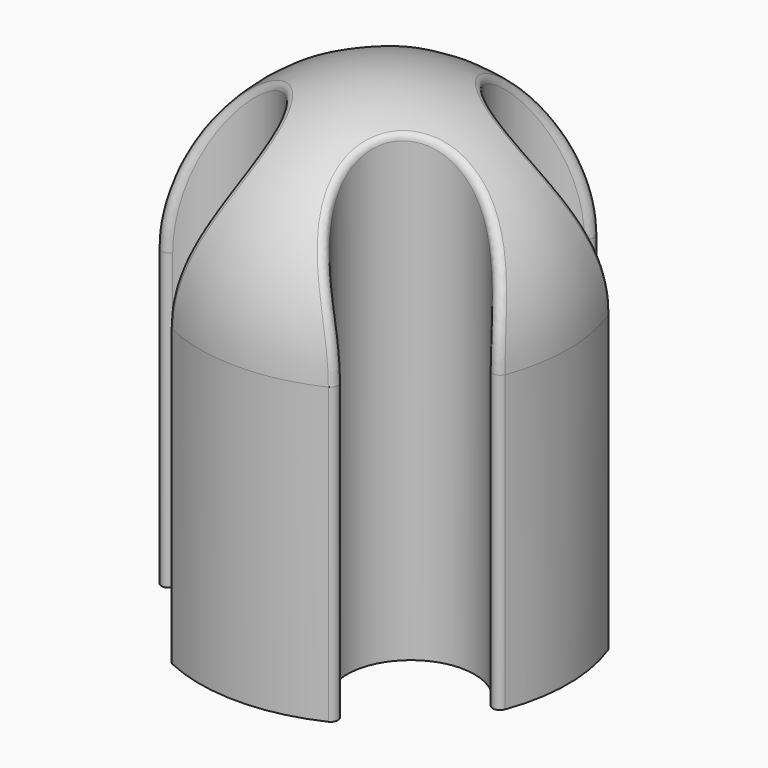
from build123d import *

# Parameters (mm, degrees)
F3_DEPTH = 16.511
F4_R     = 0.254


with BuildPart() as f1:
    # F0 (on Right) → F1 (revolve)
    with BuildSketch(Plane.YZ):
        with BuildLine():
            Line((-6.35, 0), (0, 0))
            Line((0, 0), (0, 16.51))
            ThreePointArc((0, 16.51), (-4.4901280605, 14.6501280605), (-6.35, 10.16))
            Line((-6.35, 10.16), (-6.35, 0))
        make_face()
    revolve(axis=Axis((0, 0, 8.255), (0, 0, 1)))

    # F2 (on face) → F3 (cut, through all)
    with BuildSketch(Plane(origin=(0, 0, 0), x_dir=(1, 0, 0), z_dir=(0, 0, -1))):
        with BuildLine():
            ThreePointArc((-3.2574001394, 5.4508572107), (-4.6639812108, 4.3092666737), (-5.690978087, 2.8169608469))
            ThreePointArc((-5.690978087, 2.8169608469), (-1.9306863278, 1.7838498643), (-3.2574001394, 5.4508572107))
        make_face()
        with BuildLine():
            ThreePointArc((5.690978087, 2.8169608469), (4.6639812108, 4.3092666737), (3.2574001394, 5.4508572107))
            ThreePointArc((3.2574001394, 5.4508572107), (1.9306863278, 1.7838498643), (5.690978087, 2.8169608469))
        make_face()
        with BuildLine():
            ThreePointArc((5.690978087, -2.8169608469), (1.9306863278, -1.7838498643), (3.2574001394, -5.4508572107))
            ThreePointArc((3.2574001394, -5.4508572107), (4.6639812108, -4.3092666737), (5.690978087, -2.8169608469))
        make_face()
        with BuildLine():
            ThreePointArc((-3.2574001394, -5.4508572107), (-1.9306863278, -1.7838498643), (-5.690978087, -2.8169608469))
            ThreePointArc((-5.690978087, -2.8169608469), (-4.6639812108, -4.3092666737), (-3.2574001394, -5.4508572107))
        make_face()
    extrude(amount=-F3_DEPTH, mode=Mode.SUBTRACT)

    # F4
    f4_edges = [f1.edges().sort_by_distance(p)[0] for p in [
        (-3.2574, -5.450857, 5.08),
        (3.2574, -5.450857, 5.08),
        (5.690978, 2.816961, 5.08),
        (-3.2574, 5.450857, 5.08),
    ]]
    fillet(f4_edges, radius=F4_R)


solid = f1.part
